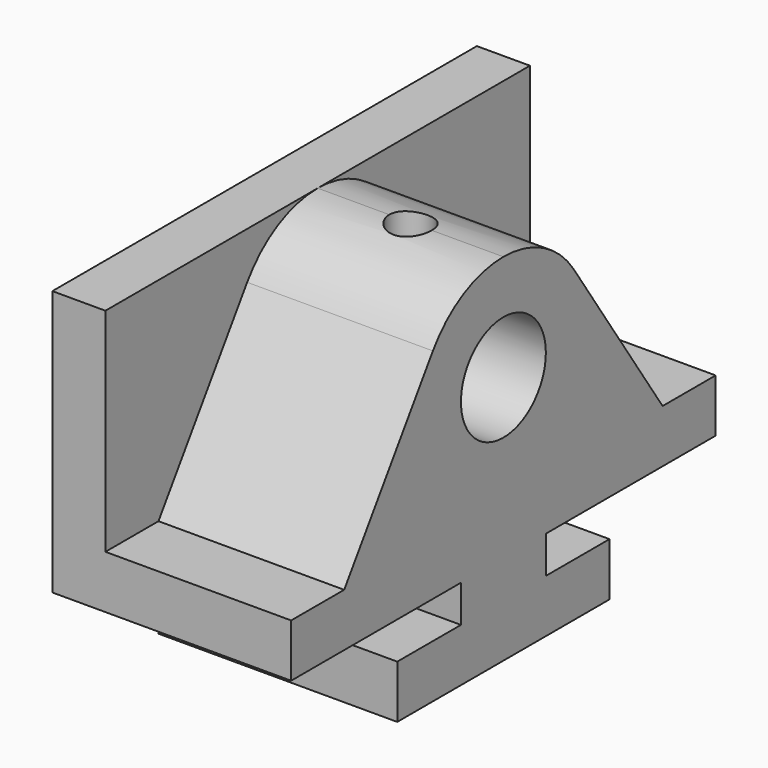
from build123d import *

# Parameters (mm, degrees)
F1_DEPTH = 57.15
F3_DEPTH = 44.45
F4_R     = 12.7
F5_DEPTH = 44.45
F8_R     = 5.08
F9_DEPTH = 25.4


with BuildPart() as f1:
    # F0 (on Right) → F1 (new body)
    with BuildSketch(Plane.YZ):
        Polygon((0, 12.7), (0, 0), (63.5, 0), (63.5, 12.7), (44.45, 12.7), (44.45, 21.59), (95.25, 21.59), (95.25, 85.09), (-31.75, 85.09), (-31.75, 21.59), (19.05, 21.59), (19.05, 12.7), align=None)
    extrude(amount=-F1_DEPTH)

    # F2 (on face) → F3 (cut)
    with BuildSketch(Plane.YZ):
        with BuildLine():
            Line((-31.75, 85.09), (-31.75, 34.29))
            Line((-31.75, 34.29), (-15.875, 34.29))
            Line((-15.875, 34.29), (10.6565743945, 73.8401730104))
            ThreePointArc((10.6565743945, 73.8401730104), (19.7970588235, 82.1017647059), (31.75, 85.09))
            Line((31.75, 85.09), (-31.75, 85.09))
        make_face()
        with BuildLine():
            Line((95.25, 85.09), (31.75, 85.09))
            ThreePointArc((31.75, 85.09), (43.7029411765, 82.1017647059), (52.8434256055, 73.8401730104))
            Line((52.8434256055, 73.8401730104), (79.375, 34.29))
            Line((79.375, 34.29), (95.25, 34.29))
            Line((95.25, 34.29), (95.25, 85.09))
        make_face()
    extrude(amount=-F3_DEPTH, mode=Mode.SUBTRACT)

    # F4 (on face) → F5 (cut)
    with BuildSketch(Plane.YZ):
        with Locations((31.75, 59.69)):
            Circle(F4_R)
    extrude(amount=-F5_DEPTH, mode=Mode.SUBTRACT)

    # F8 (on offset) → F9 (cut)
    with BuildSketch(Plane.XY.offset(85.09)):
        with Locations((-22.225, 31.75)):
            Circle(F8_R)
    extrude(amount=-F9_DEPTH, mode=Mode.SUBTRACT)


solid = f1.part
